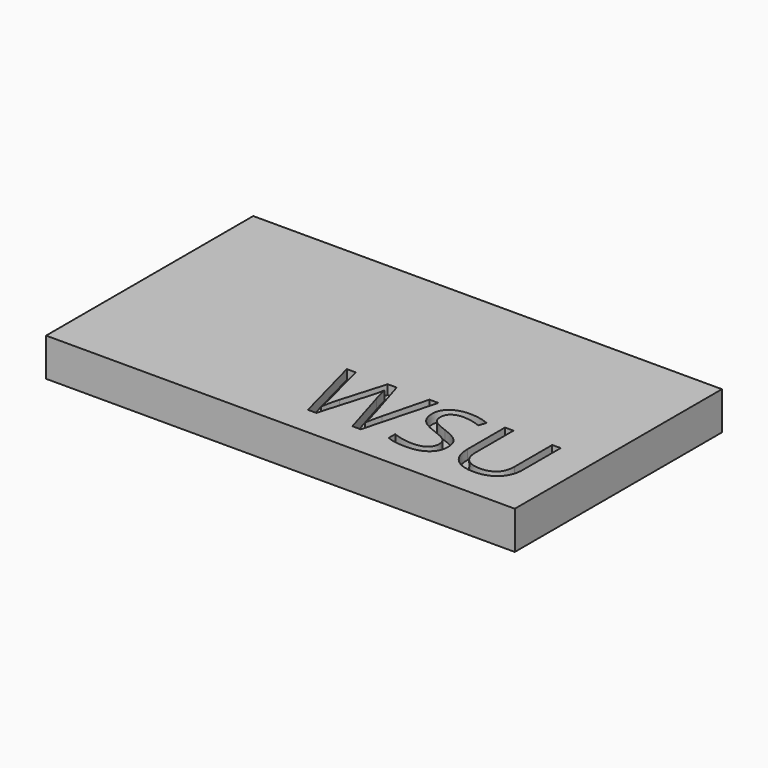
from build123d import *

# Parameters (mm, degrees)
F0_W         = 312.7297013998
F0_H         = 172.7529317141
F1_DEPTH     = 25.4
F2_TEXT_SIZE = 68.0013663239
F3_DEPTH     = 6.35


# Not quite as in the source:
# - Text() gives the source's letters only with a copy of the font that has no kerning and outlines rounded to 1/6400 em; it was checked with that copy


with BuildPart() as f1:
    # F0 (on Top) → F1 (new body)
    with BuildSketch(Plane.XY):
        with Locations((1.3875439763, -1.4350265265)):
            Rectangle(F0_W, F0_H)
    extrude(amount=F1_DEPTH)


with BuildPart() as f3:
    # F2 (on face) → F3 (new body)
    with BuildSketch(Plane.XY.offset(25.4)):
        with Locations((117.0694679022, 109.8050177097)):
            Text('WSU', F2_TEXT_SIZE, font='Open Sans', text_align=(TextAlign.LEFT, TextAlign.BOTTOM))
    extrude(amount=-F3_DEPTH)


with BuildPart() as f3_1:
    # F4: moved
    add(f3.part.moved(Location((-127, -177.8, 0))))


with BuildPart() as f1_1:
    add(f1.part)

    # F5: cut F3
    add(f3_1.part, mode=Mode.SUBTRACT)


solid = f1_1.part
